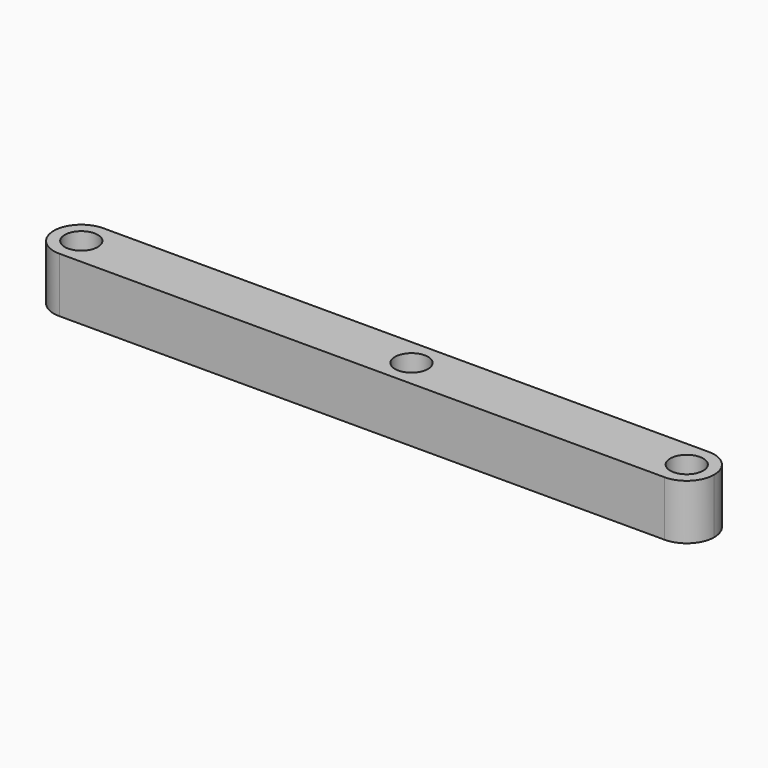
from build123d import *

# Parameters (mm, degrees)
F1_DEPTH = 5
F2_D     = 3
F3_R     = 2.49999


# Not quite as in the source:
# - a fillet or chamfer is up to 0.001 mm smaller than in the source, because OpenCascade refuses the exact size


with BuildPart() as f1:
    # F0 (on Top) → F1 (new body)
    with BuildSketch(Plane.XY):
        Polygon((43.4433006123, 0), (68.4433006123, 0), (68.4433006123, 5), (8.4433006123, 5), (8.4433006123, 0), (40.9433006123, 0), align=None)
    extrude(amount=F1_DEPTH)

    # F2 (through all)
    with Locations(Plane(origin=(0, 0, 0), x_dir=(1, 0, 0), z_dir=(0, 0, -1))):
        with Locations((40.9433006123, -2.5), (65.9433006123, -2.5), (10.9449457377, -2.5)):
            Hole(F2_D / 2)

    # F3 (radius 2.5 in the source; OpenCascade refuses exactly that, so slightly less here)
    f3_edges = [f1.edges().sort_by_distance(p)[0] for p in [
        (8.443301, 0, 2.5),
        (8.443301, 5, 2.5),
        (68.443301, 0, 2.5),
        (68.443301, 5, 2.5),
    ]]
    fillet(f3_edges, radius=F3_R)


solid = f1.part
